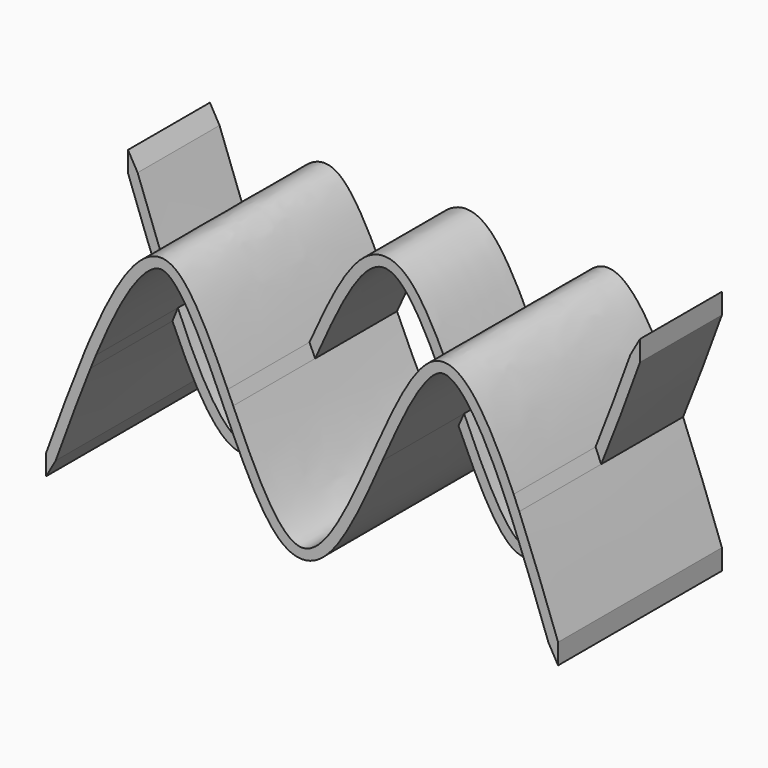
from build123d import *

# Parameters (mm, degrees)
F1_DEPTH = 25.4
F2_DEPTH = 50.8


# Not quite as in the source:
# - the dataset's text gives a spline's control points without its knots; the knots are read off the source's solid


with BuildPart() as f1:
    # F0 (on Front) → F1 (new body)
    with BuildSketch(Plane.XZ):
        with BuildLine():
            add(Edge.make_bspline(
                [(-117.3705114487, 25.4), (-116.9060848347, 26.5273856524), (-116.4416582207, 27.6335786963), (-115.9772316067, 28.715512797)],
                knots=[0.0758227445, 0.0758227445, 0.0758227445, 0.0758227445, 0.0867934519, 0.0867934519, 0.0867934519, 0.0867934519], degree=3))
            add(Edge.make_bspline(
                [(-124.6136513139, 51.6700229585), (-123.2907346472, 48.0414515299), (-120.6484437684, 40.7941401175), (-117.7726694232, 33.2147648458), (-116.2182073937, 29.3149055202), (-115.9772316067, 28.715512797)],
                knots=[0, 0, 0, 0, 0.03125, 0.0625, 0.0682366361, 0.0682366361, 0.0682366361, 0.0682366361], degree=3))
            Line((-124.6136513139, 51.6700229585), (-127, 55.88))
            Line((-127, 55.88), (-127, 50.8))
            add(Edge.make_bspline(
                [(-127, 50.8), (-123.7901704829, 41.9958961817), (-120.5803409658, 33.1917923634), (-117.3705114487, 25.4)],
                knots=[0, 0, 0, 0, 0.0758227445, 0.0758227445, 0.0758227445, 0.0758227445], degree=3))
        make_face()
    extrude(amount=F1_DEPTH)


with BuildPart() as f1b:
    # F0 (on Front) → F1, piece 2 (new body)
    with BuildSketch(Plane.XZ):
        with BuildLine():
            add(Edge.make_bspline(
                [(-115.9772316067, 22.084487203), (-109.0681544045, 5.9890137655), (-97.7362143666, -11.604355123), (-86.4042743287, 12.4028441847), (-81.981411493, 22.2836577941)],
                knots=[0.0867934519, 0.0867934519, 0.0867934519, 0.0867934519, 0.25, 0.3544770749, 0.3544770749, 0.3544770749, 0.3544770749], degree=3))
            add(Edge.make_bspline(
                [(-83.3717905897, 25.4), (-82.9091612158, 24.361974123), (-82.4457099688, 23.3209782252), (-81.981411493, 22.2836577941)],
                knots=[0.3617970411, 0.3617970411, 0.3617970411, 0.3617970411, 0.3727319162, 0.3727319162, 0.3727319162, 0.3727319162], degree=3))
            add(Edge.make_bspline(
                [(-114.6211715811, 25.4), (-114.0032712863, 23.9167755489), (-112.7325521807, 20.9477362951), (-110.8165502079, 16.7706812478), (-108.8774430943, 12.9071490359), (-106.9597149792, 9.4978455452), (-105.0772714491, 6.6065136322), (-103.2567403247, 4.300699074), (-101.548493482, 2.6470132768), (-100.3008724778, 1.8506608183), (-99.4636870621, 1.527482946), (-98.9132376363, 1.4140252539), (-98.412065553, 1.4032244512), (-97.9073076465, 1.4873351716), (-97.3448464442, 1.6924896347), (-96.7027500118, 2.0588940516), (-95.9628056471, 2.6408018611), (-95.1415705548, 3.4526098059), (-94.2701356609, 4.4767729227), (-93.062163993, 6.1026096637), (-91.4956057417, 8.5743632039), (-89.5715929579, 12.0978457012), (-87.6224014858, 16.0441304349), (-85.6573674341, 20.2861774401), (-84.2374898585, 23.457996584), (-83.47426157, 25.1700804679), (-83.3717905897, 25.4)],
                knots=[0.0790085188, 0.0790085188, 0.0790085188, 0.0790085188, 0.09375, 0.109375, 0.125, 0.140625, 0.15625, 0.171875, 0.1875, 0.203125, 0.2109375, 0.21875, 0.2265625, 0.234375, 0.2421875, 0.25, 0.2578125, 0.265625, 0.2734375, 0.28125, 0.296875, 0.3125, 0.328125, 0.34375, 0.359375, 0.3617970411, 0.3617970411, 0.3617970411, 0.3617970411], degree=3))
            add(Edge.make_bspline(
                [(-115.9772316067, 22.084487203), (-115.5247429283, 23.2099879205), (-115.0726831632, 24.3161794805), (-114.6211715811, 25.4)],
                knots=[0.0682366361, 0.0682366361, 0.0682366361, 0.0682366361, 0.0790085188, 0.0790085188, 0.0790085188, 0.0790085188], degree=3))
        make_face()
    extrude(amount=F1_DEPTH)


with BuildPart() as f1c:
    # F0 (on Front) → F1, piece 3 (new body)
    with BuildSketch(Plane.XZ):
        with BuildLine():
            add(Edge.make_bspline(
                [(-80.5910012785, 25.4), (-74.8940008523, 38.1827567283), (-69.1970004262, 50.8), (-63.5, 50.8)],
                knots=[0.3654251868, 0.3654251868, 0.3654251868, 0.3654251868, 0.5, 0.5, 0.5, 0.5], degree=3))
            add(Edge.make_bspline(
                [(-63.5, 50.8), (-57.8029995738, 50.8), (-52.1059991477, 38.1827567283), (-46.4089987215, 25.4)],
                knots=[0.5, 0.5, 0.5, 0.5, 0.6345748132, 0.6345748132, 0.6345748132, 0.6345748132], degree=3))
            add(Edge.make_bspline(
                [(-46.4089987215, 25.4), (-45.94552865, 26.4399200863), (-45.4820585785, 27.4809356016), (-45.018588507, 28.5163422059)],
                knots=[0.6345748132, 0.6345748132, 0.6345748132, 0.6345748132, 0.6455229251, 0.6455229251, 0.6455229251, 0.6455229251], degree=3))
            add(Edge.make_bspline(
                [(-81.981411493, 28.5163422059), (-81.8851078934, 28.7315005505), (-81.1250739845, 30.4276534817), (-79.6970703406, 33.5796101949), (-77.6868856038, 37.8122350706), (-75.657530467, 41.7598232703), (-73.5958588427, 45.3184849529), (-71.8283108694, 47.8812173235), (-70.3498547959, 49.6480159512), (-69.1914352087, 50.8206698204), (-67.9584485225, 51.8259451611), (-66.6165749521, 52.6365741471), (-65.3777704052, 53.1030958043), (-64.3198290774, 53.3045943231), (-63.5, 53.3577028384), (-62.6801709226, 53.3045943231), (-61.6222295948, 53.1030958043), (-60.3834250479, 52.6365741471), (-59.0415514775, 51.8259451611), (-57.8085647913, 50.8206698204), (-56.6501452041, 49.6480159512), (-55.1716891306, 47.8812173235), (-53.4041411573, 45.3184849529), (-51.342469533, 41.7598232703), (-49.3131143962, 37.8122350706), (-47.3029296594, 33.5796101949), (-45.8749260155, 30.4276534817), (-45.1148921066, 28.7315005505), (-45.018588507, 28.5163422059)],
                knots=[0.3727319162, 0.3727319162, 0.3727319162, 0.3727319162, 0.375, 0.390625, 0.40625, 0.421875, 0.4375, 0.453125, 0.4609375, 0.46875, 0.4765625, 0.484375, 0.4921875, 0.49609375, 0.5, 0.50390625, 0.5078125, 0.515625, 0.5234375, 0.53125, 0.5390625, 0.546875, 0.5625, 0.578125, 0.59375, 0.609375, 0.625, 0.6272680838, 0.6272680838, 0.6272680838, 0.6272680838], degree=3))
            add(Edge.make_bspline(
                [(-81.981411493, 28.5163422059), (-81.5179414215, 27.4809356016), (-81.05447135, 26.4399200863), (-80.5910012785, 25.4)],
                knots=[0.3544770749, 0.3544770749, 0.3544770749, 0.3544770749, 0.3654251868, 0.3654251868, 0.3654251868, 0.3654251868], degree=3))
        make_face()
    extrude(amount=F1_DEPTH)


with BuildPart() as f1d:
    # F0 (on Front) → F1, piece 4 (new body)
    with BuildSketch(Plane.XZ):
        with BuildLine():
            add(Edge.make_bspline(
                [(-45.018588507, 22.2836577941), (-44.5542900312, 23.3209782252), (-44.0908387842, 24.361974123), (-43.6282094103, 25.4)],
                knots=[0.6272680838, 0.6272680838, 0.6272680838, 0.6272680838, 0.6382029589, 0.6382029589, 0.6382029589, 0.6382029589], degree=3))
            add(Edge.make_bspline(
                [(-45.018588507, 22.2836577941), (-40.5957256713, 12.4028441847), (-29.2637856334, -11.604355123), (-17.9318455955, 5.9890137655), (-11.0227683933, 22.084487203)],
                knots=[0.6455229251, 0.6455229251, 0.6455229251, 0.6455229251, 0.75, 0.9132065481, 0.9132065481, 0.9132065481, 0.9132065481], degree=3))
            add(Edge.make_bspline(
                [(-12.3788284189, 25.4), (-11.9273168368, 24.3161794805), (-11.4752570717, 23.2099879205), (-11.0227683933, 22.084487203)],
                knots=[0.9209914812, 0.9209914812, 0.9209914812, 0.9209914812, 0.9317633639, 0.9317633639, 0.9317633639, 0.9317633639], degree=3))
            add(Edge.make_bspline(
                [(-43.6282094103, 25.4), (-43.52573843, 25.1700804679), (-42.7625101415, 23.457996584), (-41.3426325659, 20.2861774401), (-39.3775985142, 16.0441304349), (-37.4284070421, 12.0978457012), (-35.5043942583, 8.5743632039), (-33.937836007, 6.1026096637), (-32.7298643391, 4.4767729227), (-31.8584294452, 3.4526098059), (-31.0371943529, 2.6408018611), (-30.2972499882, 2.0588940516), (-29.6551535558, 1.6924896347), (-29.0926923535, 1.4873351716), (-28.587934447, 1.4032244512), (-28.0867623637, 1.4140252539), (-27.5363129379, 1.527482946), (-26.6991275222, 1.8506608183), (-25.451506518, 2.6470132768), (-23.7432596753, 4.300699074), (-21.9227285509, 6.6065136322), (-20.0402850208, 9.4978455452), (-18.1225569057, 12.9071490359), (-16.1834497921, 16.7706812478), (-14.2674478194, 20.9477362951), (-12.9967287137, 23.9167755489), (-12.3788284189, 25.4)],
                knots=[0.6382029589, 0.6382029589, 0.6382029589, 0.6382029589, 0.640625, 0.65625, 0.671875, 0.6875, 0.703125, 0.71875, 0.7265625, 0.734375, 0.7421875, 0.75, 0.7578125, 0.765625, 0.7734375, 0.78125, 0.7890625, 0.796875, 0.8125, 0.828125, 0.84375, 0.859375, 0.875, 0.890625, 0.90625, 0.9209914812, 0.9209914812, 0.9209914812, 0.9209914812], degree=3))
        make_face()
    extrude(amount=F1_DEPTH)


with BuildPart() as f1e:
    # F0 (on Front) → F1, piece 5 (new body)
    with BuildSketch(Plane.XZ):
        with BuildLine():
            add(Edge.make_bspline(
                [(-11.0227683933, 28.715512797), (-10.7817926063, 29.3149055202), (-9.2273305768, 33.2147648458), (-6.3515562316, 40.7941401175), (-3.7092653528, 48.0414515299), (-2.3863486861, 51.6700229585)],
                knots=[0.9317633639, 0.9317633639, 0.9317633639, 0.9317633639, 0.9375, 0.96875, 1, 1, 1, 1], degree=3))
            add(Edge.make_bspline(
                [(-11.0227683933, 28.715512797), (-10.5583417793, 27.6335786963), (-10.0939151653, 26.5273856524), (-9.6294885513, 25.4)],
                knots=[0.9132065481, 0.9132065481, 0.9132065481, 0.9132065481, 0.9241772555, 0.9241772555, 0.9241772555, 0.9241772555], degree=3))
            add(Edge.make_bspline(
                [(-9.6294885513, 25.4), (-6.4196590342, 33.1917923634), (-3.2098295171, 41.9958961817), (0, 50.8)],
                knots=[0.9241772555, 0.9241772555, 0.9241772555, 0.9241772555, 1, 1, 1, 1], degree=3))
            Line((0, 50.8), (0, 55.88))
            Line((0, 55.88), (-2.3863486861, 51.6700229585))
        make_face()
    extrude(amount=F1_DEPTH)


with BuildPart() as f2:
    # F0 (on Front) → F2 (new body)
    with BuildSketch(Plane.XZ):
        with BuildLine():
            add(Edge.make_bspline(
                [(-124.6136513139, -0.8700229585), (-123.2907346472, 2.7585484701), (-120.6484437684, 10.0058598825), (-117.7726694232, 17.5852351542), (-116.2182073937, 21.4850944798), (-115.9772316067, 22.084487203)],
                knots=[0, 0, 0, 0, 0.03125, 0.0625, 0.0682366361, 0.0682366361, 0.0682366361, 0.0682366361], degree=3))
            add(Edge.make_bspline(
                [(-117.3705114487, 25.4), (-116.9060848347, 24.2726143476), (-116.4416582207, 23.1664213037), (-115.9772316067, 22.084487203)],
                knots=[0.0758227445, 0.0758227445, 0.0758227445, 0.0758227445, 0.0867934519, 0.0867934519, 0.0867934519, 0.0867934519], degree=3))
            add(Edge.make_bspline(
                [(-127, 0), (-123.7901704829, 8.8041038183), (-120.5803409658, 17.6082076366), (-117.3705114487, 25.4)],
                knots=[0, 0, 0, 0, 0.0758227445, 0.0758227445, 0.0758227445, 0.0758227445], degree=3))
            Line((-127, 0), (-127, -5.08))
            Line((-127, -5.08), (-124.6136513139, -0.8700229585))
        make_face()
        with BuildLine():
            add(Edge.make_bspline(
                [(-115.9772316067, 28.715512797), (-115.5247429283, 27.5900120795), (-115.0726831632, 26.4838205195), (-114.6211715811, 25.4)],
                knots=[0.0682366361, 0.0682366361, 0.0682366361, 0.0682366361, 0.0790085188, 0.0790085188, 0.0790085188, 0.0790085188], degree=3))
            add(Edge.make_bspline(
                [(-117.3705114487, 25.4), (-116.9060848347, 26.5273856524), (-116.4416582207, 27.6335786963), (-115.9772316067, 28.715512797)],
                knots=[0.0758227445, 0.0758227445, 0.0758227445, 0.0758227445, 0.0867934519, 0.0867934519, 0.0867934519, 0.0867934519], degree=3))
            add(Edge.make_bspline(
                [(-117.3705114487, 25.4), (-116.9060848347, 24.2726143476), (-116.4416582207, 23.1664213037), (-115.9772316067, 22.084487203)],
                knots=[0.0758227445, 0.0758227445, 0.0758227445, 0.0758227445, 0.0867934519, 0.0867934519, 0.0867934519, 0.0867934519], degree=3))
            add(Edge.make_bspline(
                [(-115.9772316067, 22.084487203), (-115.5247429283, 23.2099879205), (-115.0726831632, 24.3161794805), (-114.6211715811, 25.4)],
                knots=[0.0682366361, 0.0682366361, 0.0682366361, 0.0682366361, 0.0790085188, 0.0790085188, 0.0790085188, 0.0790085188], degree=3))
        make_face()
        with BuildLine():
            add(Edge.make_bspline(
                [(-83.3717905897, 25.4), (-82.9091612158, 26.438025877), (-82.4457099688, 27.4790217748), (-81.981411493, 28.5163422059)],
                knots=[0.3617970411, 0.3617970411, 0.3617970411, 0.3617970411, 0.3727319162, 0.3727319162, 0.3727319162, 0.3727319162], degree=3))
            add(Edge.make_bspline(
                [(-115.9772316067, 28.715512797), (-109.0681544045, 44.8109862345), (-97.7362143666, 62.404355123), (-86.4042743287, 38.3971558153), (-81.981411493, 28.5163422059)],
                knots=[0.0867934519, 0.0867934519, 0.0867934519, 0.0867934519, 0.25, 0.3544770749, 0.3544770749, 0.3544770749, 0.3544770749], degree=3))
            add(Edge.make_bspline(
                [(-115.9772316067, 28.715512797), (-115.5247429283, 27.5900120795), (-115.0726831632, 26.4838205195), (-114.6211715811, 25.4)],
                knots=[0.0682366361, 0.0682366361, 0.0682366361, 0.0682366361, 0.0790085188, 0.0790085188, 0.0790085188, 0.0790085188], degree=3))
            add(Edge.make_bspline(
                [(-114.6211715811, 25.4), (-114.0032712862, 26.8832244512), (-112.7325521806, 29.8522637049), (-110.8165502079, 34.0293187522), (-108.8774430943, 37.8928509641), (-106.9597149792, 41.3021544548), (-105.0772714491, 44.1934863678), (-103.2567403247, 46.499300926), (-101.548493482, 48.1529867232), (-100.3008724778, 48.9493391817), (-99.4636870621, 49.272517054), (-98.9132376363, 49.3859747461), (-98.412065553, 49.3967755488), (-97.9073076465, 49.3126648284), (-97.3448464442, 49.1075103653), (-96.7027500118, 48.7411059484), (-95.9628056471, 48.1591981389), (-95.1415705548, 47.3473901941), (-94.2701356609, 46.3232270773), (-93.062163993, 44.6973903363), (-91.4956057417, 42.2256367961), (-89.5715929579, 38.7021542988), (-87.6224014858, 34.7558695651), (-85.6573674341, 30.5138225599), (-84.2374898585, 27.342003416), (-83.47426157, 25.6299195321), (-83.3717905897, 25.4)],
                knots=[0.0790085188, 0.0790085188, 0.0790085188, 0.0790085188, 0.09375, 0.109375, 0.125, 0.140625, 0.15625, 0.171875, 0.1875, 0.203125, 0.2109375, 0.21875, 0.2265625, 0.234375, 0.2421875, 0.25, 0.2578125, 0.265625, 0.2734375, 0.28125, 0.296875, 0.3125, 0.328125, 0.34375, 0.359375, 0.3617970411, 0.3617970411, 0.3617970411, 0.3617970411], degree=3))
        make_face()
        with BuildLine():
            add(Edge.make_bspline(
                [(-81.981411493, 22.2836577941), (-81.5179414215, 23.3190643984), (-81.05447135, 24.3600799137), (-80.5910012785, 25.4)],
                knots=[0.3544770749, 0.3544770749, 0.3544770749, 0.3544770749, 0.3654251868, 0.3654251868, 0.3654251868, 0.3654251868], degree=3))
            add(Edge.make_bspline(
                [(-81.981411493, 28.5163422059), (-81.5179414215, 27.4809356016), (-81.05447135, 26.4399200863), (-80.5910012785, 25.4)],
                knots=[0.3544770749, 0.3544770749, 0.3544770749, 0.3544770749, 0.3654251868, 0.3654251868, 0.3654251868, 0.3654251868], degree=3))
            add(Edge.make_bspline(
                [(-83.3717905897, 25.4), (-82.9091612158, 26.438025877), (-82.4457099688, 27.4790217748), (-81.981411493, 28.5163422059)],
                knots=[0.3617970411, 0.3617970411, 0.3617970411, 0.3617970411, 0.3727319162, 0.3727319162, 0.3727319162, 0.3727319162], degree=3))
            add(Edge.make_bspline(
                [(-83.3717905897, 25.4), (-82.9091612158, 24.361974123), (-82.4457099688, 23.3209782252), (-81.981411493, 22.2836577941)],
                knots=[0.3617970411, 0.3617970411, 0.3617970411, 0.3617970411, 0.3727319162, 0.3727319162, 0.3727319162, 0.3727319162], degree=3))
        make_face()
        with BuildLine():
            add(Edge.make_bspline(
                [(-63.5, 0), (-57.8029995738, 0), (-52.1059991477, 12.6172432717), (-46.4089987215, 25.4)],
                knots=[0.5, 0.5, 0.5, 0.5, 0.6345748132, 0.6345748132, 0.6345748132, 0.6345748132], degree=3))
            add(Edge.make_bspline(
                [(-80.5910012785, 25.4), (-74.8940008523, 12.6172432717), (-69.1970004262, 0), (-63.5, 0)],
                knots=[0.3654251868, 0.3654251868, 0.3654251868, 0.3654251868, 0.5, 0.5, 0.5, 0.5], degree=3))
            add(Edge.make_bspline(
                [(-81.981411493, 22.2836577941), (-81.5179414215, 23.3190643984), (-81.05447135, 24.3600799137), (-80.5910012785, 25.4)],
                knots=[0.3544770749, 0.3544770749, 0.3544770749, 0.3544770749, 0.3654251868, 0.3654251868, 0.3654251868, 0.3654251868], degree=3))
            add(Edge.make_bspline(
                [(-81.981411493, 22.2836577941), (-81.8851078934, 22.0684994495), (-81.1250739845, 20.3723465183), (-79.6970703406, 17.2203898051), (-77.6868856038, 12.9877649294), (-75.657530467, 9.0401767297), (-73.5958588427, 5.4815150471), (-71.8283108694, 2.9187826765), (-70.3498547959, 1.1519840488), (-69.1914352087, -0.0206698204), (-67.9584485225, -1.0259451611), (-66.6165749521, -1.8365741471), (-65.3777704052, -2.3030958043), (-64.3198290774, -2.5045943231), (-63.5, -2.5577028384), (-62.6801709226, -2.5045943231), (-61.6222295948, -2.3030958043), (-60.3834250479, -1.8365741471), (-59.0415514775, -1.0259451611), (-57.8085647913, -0.0206698204), (-56.6501452041, 1.1519840488), (-55.1716891306, 2.9187826765), (-53.4041411573, 5.4815150471), (-51.342469533, 9.0401767297), (-49.3131143962, 12.9877649294), (-47.3029296594, 17.2203898051), (-45.8749260155, 20.3723465183), (-45.1148921066, 22.0684994495), (-45.018588507, 22.2836577941)],
                knots=[0.3727319162, 0.3727319162, 0.3727319162, 0.3727319162, 0.375, 0.390625, 0.40625, 0.421875, 0.4375, 0.453125, 0.4609375, 0.46875, 0.4765625, 0.484375, 0.4921875, 0.49609375, 0.5, 0.50390625, 0.5078125, 0.515625, 0.5234375, 0.53125, 0.5390625, 0.546875, 0.5625, 0.578125, 0.59375, 0.609375, 0.625, 0.6272680838, 0.6272680838, 0.6272680838, 0.6272680838], degree=3))
            add(Edge.make_bspline(
                [(-46.4089987215, 25.4), (-45.94552865, 24.3600799137), (-45.4820585785, 23.3190643984), (-45.018588507, 22.2836577941)],
                knots=[0.6345748132, 0.6345748132, 0.6345748132, 0.6345748132, 0.6455229251, 0.6455229251, 0.6455229251, 0.6455229251], degree=3))
        make_face()
        with BuildLine():
            add(Edge.make_bspline(
                [(-46.4089987215, 25.4), (-45.94552865, 26.4399200863), (-45.4820585785, 27.4809356016), (-45.018588507, 28.5163422059)],
                knots=[0.6345748132, 0.6345748132, 0.6345748132, 0.6345748132, 0.6455229251, 0.6455229251, 0.6455229251, 0.6455229251], degree=3))
            add(Edge.make_bspline(
                [(-46.4089987215, 25.4), (-45.94552865, 24.3600799137), (-45.4820585785, 23.3190643984), (-45.018588507, 22.2836577941)],
                knots=[0.6345748132, 0.6345748132, 0.6345748132, 0.6345748132, 0.6455229251, 0.6455229251, 0.6455229251, 0.6455229251], degree=3))
            add(Edge.make_bspline(
                [(-45.018588507, 22.2836577941), (-44.5542900312, 23.3209782252), (-44.0908387842, 24.361974123), (-43.6282094103, 25.4)],
                knots=[0.6272680838, 0.6272680838, 0.6272680838, 0.6272680838, 0.6382029589, 0.6382029589, 0.6382029589, 0.6382029589], degree=3))
            add(Edge.make_bspline(
                [(-45.018588507, 28.5163422059), (-44.5542900312, 27.4790217748), (-44.0908387842, 26.438025877), (-43.6282094103, 25.4)],
                knots=[0.6272680838, 0.6272680838, 0.6272680838, 0.6272680838, 0.6382029589, 0.6382029589, 0.6382029589, 0.6382029589], degree=3))
        make_face()
        with BuildLine():
            add(Edge.make_bspline(
                [(-45.018588507, 28.5163422059), (-40.5957256713, 38.3971558153), (-29.2637856334, 62.404355123), (-17.9318455955, 44.8109862345), (-11.0227683933, 28.715512797)],
                knots=[0.6455229251, 0.6455229251, 0.6455229251, 0.6455229251, 0.75, 0.9132065481, 0.9132065481, 0.9132065481, 0.9132065481], degree=3))
            add(Edge.make_bspline(
                [(-45.018588507, 28.5163422059), (-44.5542900312, 27.4790217748), (-44.0908387842, 26.438025877), (-43.6282094103, 25.4)],
                knots=[0.6272680838, 0.6272680838, 0.6272680838, 0.6272680838, 0.6382029589, 0.6382029589, 0.6382029589, 0.6382029589], degree=3))
            add(Edge.make_bspline(
                [(-43.6282094103, 25.4), (-43.52573843, 25.6299195321), (-42.7625101415, 27.342003416), (-41.3426325659, 30.5138225599), (-39.3775985142, 34.7558695651), (-37.4284070421, 38.7021542988), (-35.5043942583, 42.2256367961), (-33.937836007, 44.6973903363), (-32.7298643391, 46.3232270773), (-31.8584294452, 47.3473901941), (-31.0371943529, 48.1591981389), (-30.2972499882, 48.7411059484), (-29.6551535558, 49.1075103653), (-29.0926923535, 49.3126648284), (-28.587934447, 49.3967755488), (-28.0867623637, 49.3859747461), (-27.5363129379, 49.272517054), (-26.6991275222, 48.9493391817), (-25.451506518, 48.1529867232), (-23.7432596753, 46.499300926), (-21.9227285509, 44.1934863678), (-20.0402850208, 41.3021544548), (-18.1225569057, 37.8928509641), (-16.1834497921, 34.0293187522), (-14.2674478194, 29.8522637049), (-12.9967287138, 26.8832244512), (-12.3788284189, 25.4)],
                knots=[0.6382029589, 0.6382029589, 0.6382029589, 0.6382029589, 0.640625, 0.65625, 0.671875, 0.6875, 0.703125, 0.71875, 0.7265625, 0.734375, 0.7421875, 0.75, 0.7578125, 0.765625, 0.7734375, 0.78125, 0.7890625, 0.796875, 0.8125, 0.828125, 0.84375, 0.859375, 0.875, 0.890625, 0.90625, 0.9209914812, 0.9209914812, 0.9209914812, 0.9209914812], degree=3))
            add(Edge.make_bspline(
                [(-12.3788284189, 25.4), (-11.9273168368, 26.4838205195), (-11.4752570717, 27.5900120795), (-11.0227683933, 28.715512797)],
                knots=[0.9209914812, 0.9209914812, 0.9209914812, 0.9209914812, 0.9317633639, 0.9317633639, 0.9317633639, 0.9317633639], degree=3))
        make_face()
        with BuildLine():
            add(Edge.make_bspline(
                [(-11.0227683933, 28.715512797), (-10.5583417793, 27.6335786963), (-10.0939151653, 26.5273856524), (-9.6294885513, 25.4)],
                knots=[0.9132065481, 0.9132065481, 0.9132065481, 0.9132065481, 0.9241772555, 0.9241772555, 0.9241772555, 0.9241772555], degree=3))
            add(Edge.make_bspline(
                [(-12.3788284189, 25.4), (-11.9273168368, 26.4838205195), (-11.4752570717, 27.5900120795), (-11.0227683933, 28.715512797)],
                knots=[0.9209914812, 0.9209914812, 0.9209914812, 0.9209914812, 0.9317633639, 0.9317633639, 0.9317633639, 0.9317633639], degree=3))
            add(Edge.make_bspline(
                [(-12.3788284189, 25.4), (-11.9273168368, 24.3161794805), (-11.4752570717, 23.2099879205), (-11.0227683933, 22.084487203)],
                knots=[0.9209914812, 0.9209914812, 0.9209914812, 0.9209914812, 0.9317633639, 0.9317633639, 0.9317633639, 0.9317633639], degree=3))
            add(Edge.make_bspline(
                [(-11.0227683933, 22.084487203), (-10.5583417793, 23.1664213037), (-10.0939151653, 24.2726143476), (-9.6294885513, 25.4)],
                knots=[0.9132065481, 0.9132065481, 0.9132065481, 0.9132065481, 0.9241772555, 0.9241772555, 0.9241772555, 0.9241772555], degree=3))
        make_face()
        with BuildLine():
            add(Edge.make_bspline(
                [(-11.0227683933, 22.084487203), (-10.5583417793, 23.1664213037), (-10.0939151653, 24.2726143476), (-9.6294885513, 25.4)],
                knots=[0.9132065481, 0.9132065481, 0.9132065481, 0.9132065481, 0.9241772555, 0.9241772555, 0.9241772555, 0.9241772555], degree=3))
            add(Edge.make_bspline(
                [(-11.0227683933, 22.084487203), (-10.7817926063, 21.4850944798), (-9.2273305768, 17.5852351542), (-6.3515562316, 10.0058598825), (-3.7092653528, 2.7585484701), (-2.3863486861, -0.8700229585)],
                knots=[0.9317633639, 0.9317633639, 0.9317633639, 0.9317633639, 0.9375, 0.96875, 1, 1, 1, 1], degree=3))
            Line((-2.3863486861, -0.8700229585), (0, -5.08))
            Line((0, -5.08), (0, 0))
            add(Edge.make_bspline(
                [(-9.6294885513, 25.4), (-6.4196590342, 17.6082076366), (-3.2098295171, 8.8041038183), (0, 0)],
                knots=[0.9241772555, 0.9241772555, 0.9241772555, 0.9241772555, 1, 1, 1, 1], degree=3))
        make_face()
    extrude(amount=F2_DEPTH)


solid = Compound([f1.part, f1b.part, f1c.part, f1d.part, f1e.part, f2.part])
